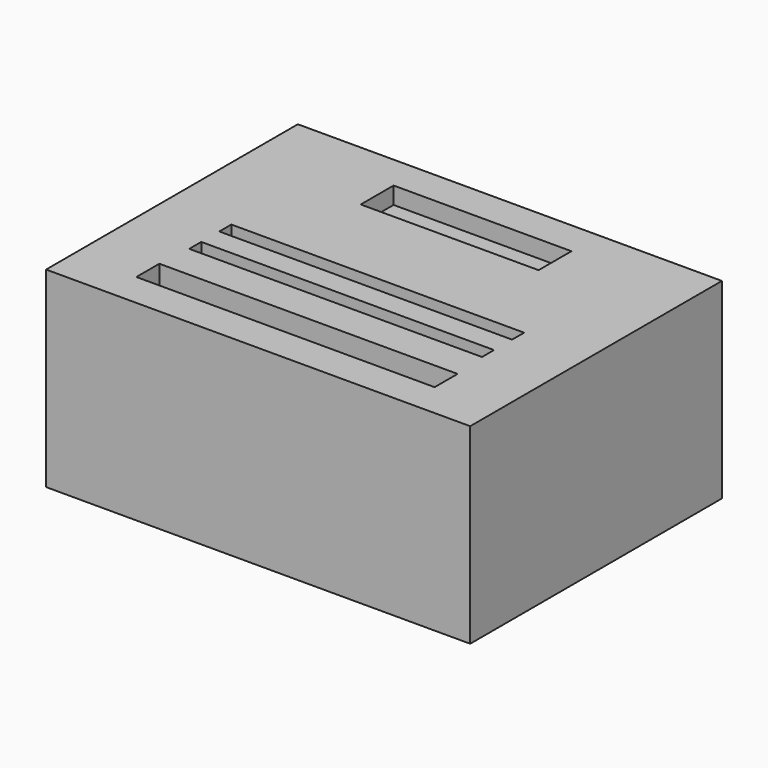
from build123d import *

# Parameters (mm, degrees)
F0_W     = 620
F0_H     = 460
F0_W_2   = 428
F0_H_2   = 22
F0_W_3   = 436
F0_H_3   = 42
F1_DEPTH = 280
F2_DEPTH = 250
F3_DEPTH = 140
F4_W     = 260
F4_H     = 60
F5_DEPTH = 25


# Not quite as in the source:
# - a feature names something its author has since deleted; it is built from what else it names


with BuildPart() as f1:
    # F0 (on Top) → F1 (new body)
    with BuildSketch(Plane.XY):
        with Locations((0.344911406, 88)):
            Rectangle(F0_W, F0_H)
        with Locations((0, 11)):
            Rectangle(F0_W_2, F0_H_2, mode=Mode.SUBTRACT)
        with Locations((0, 66)):
            Rectangle(F0_W_2, F0_H_2, mode=Mode.SUBTRACT)
        with Locations((0.344911406, -71)):
            Rectangle(F0_W_3, F0_H_3, mode=Mode.SUBTRACT)
        with Locations((0.344911406, -71)):
            Rectangle(F0_W_3, F0_H_3)
        with Locations((0, 11)):
            Rectangle(F0_W_2, F0_H_2)
        with Locations((0, 66)):
            Rectangle(F0_W_2, F0_H_2)
    extrude(amount=-F1_DEPTH)

    # F0 (on Top) → F2 (cut)
    with BuildSketch(Plane.XY):
        with Locations((0.344911406, -71)):
            Rectangle(F0_W_3, F0_H_3)
    extrude(amount=-F2_DEPTH, mode=Mode.SUBTRACT)

    # F0 (on Top) → F3 (cut)
    with BuildSketch(Plane.XY):
        with Locations((0, 11)):
            Rectangle(F0_W_2, F0_H_2)
        with Locations((0, 66)):
            Rectangle(F0_W_2, F0_H_2)
    extrude(amount=-F3_DEPTH, mode=Mode.SUBTRACT)

    # F4 (on face) → F5 (cut)
    with BuildSketch(Plane.XY):
        with Locations((0.344911406, 238)):
            Rectangle(F4_W, F4_H)
    extrude(amount=-F5_DEPTH, mode=Mode.SUBTRACT)


solid = f1.part
